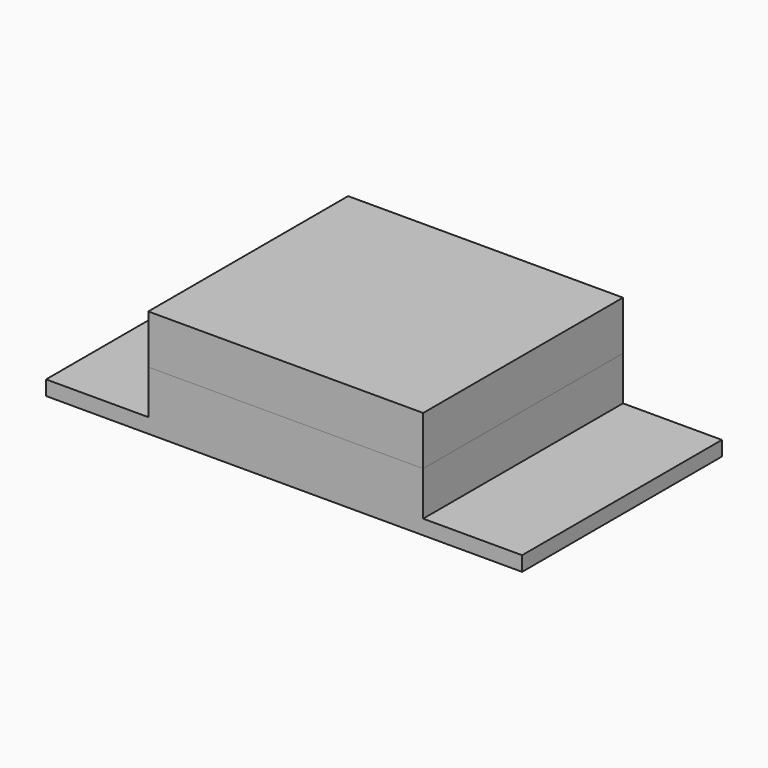
from build123d import *

# Parameters (mm, degrees)
F0_W     = 9.1
F0_H     = 23.5
F1_DEPTH = 1.5
F0_W_2   = 9.4355237663
F0_W_3   = 12.3644762337
F0_H_2   = 11.25
F2_DEPTH = 0.5
F0_W_4   = 12.7
F0_W_5   = 27.0644762337
F0_H_3   = 24.5
F3_DEPTH = 6
F4_DEPTH = 10
F5_W     = 28.0644762337
F5_H     = 25.5
F5_W_2   = 27.0644762337
F5_H_2   = 24.5
F6_DEPTH = 4
F7_W     = 28.0644762337
F7_H     = 25.5
F8_DEPTH = 1


# Not quite as in the source:
# - a feature names something its author has since deleted; it is built from what else it names


with BuildPart() as f1:
    # F0 (on Top) → F1 (new body)
    with BuildSketch(Plane.XY):
        with Locations((18.75, 0)):
            Rectangle(F0_W, F0_H)
        Polygon((24.3, -12.75), (24.3, 12.75), (14.2, 12.75), (14.2, 11.75), (23.3, 11.75), (23.3, -11.75), (14.2, -11.75), (14.2, -12.75), align=None)
    extrude(amount=F1_DEPTH)



with BuildPart() as f1b:
    # F0 (on Top) → F1, piece 2 (new body)
    with BuildSketch(Plane.XY):
        Polygon((-13.8644762337, 11.75), (-13.8644762337, 12.75), (-24.3, 12.75), (-24.3, -12.75), (-13.8644762337, -12.75), (-13.8644762337, -11.75), (-23.3, -11.75), (-23.3, 11.75), align=None)
        with Locations((-18.5822381169, 0)):
            Rectangle(F0_W_2, F0_H)
    extrude(amount=F1_DEPTH)


with BuildPart() as f2:
    # F0 (on Top) → F2 (new body)
    with BuildSketch(Plane.XY):
        with Locations((-6.6822381169, 6.125)):
            Rectangle(F0_W_3, F0_H_2)
    extrude(amount=F2_DEPTH)


with BuildPart() as f2b:
    # F0 (on Top) → F2, piece 2 (new body)
    with BuildSketch(Plane.XY):
        with Locations((6.85, 6.125)):
            Rectangle(F0_W_4, F0_H_2)
    extrude(amount=F2_DEPTH)


with BuildPart() as f2c:
    # F0 (on Top) → F2, piece 3 (new body)
    with BuildSketch(Plane.XY):
        with Locations((-6.6822381169, -6.125)):
            Rectangle(F0_W_3, F0_H_2)
    extrude(amount=F2_DEPTH)


with BuildPart() as f2d:
    # F0 (on Top) → F2, piece 4 (new body)
    with BuildSketch(Plane.XY):
        with Locations((6.85, -6.125)):
            Rectangle(F0_W_4, F0_H_2)
    extrude(amount=F2_DEPTH)


with BuildPart() as f1_1:
    add(f1.part)

    add(f1b.part)  # F3 merges F1b
    # F0 (on Top) → F3 (join)
    with BuildSketch(Plane.XY):
        Polygon((14.2, 11.75), (14.2, 12.75), (-13.8644762337, 12.75), (-13.8644762337, 11.75), (-13.8644762337, -11.75), (-13.8644762337, -12.75), (14.2, -12.75), (14.2, -11.75), align=None)
        with Locations((0.1677618831, 0)):
            Rectangle(F0_W_5, F0_H_3, mode=Mode.SUBTRACT)
    extrude(amount=F3_DEPTH)


    add(f2.part)  # F4 merges F2

    add(f2b.part)  # F4 merges F2b

    add(f2c.part)  # F4 merges F2c

    add(f2d.part)  # F4 merges F2d
    # F0 (on Top) → F4 (join)
    with BuildSketch(Plane.XY):
        with Locations((0.1677618831, 0)):
            Rectangle(F0_W_5, F0_H_3)
        with Locations((-6.6822381169, -6.125)):
            Rectangle(F0_W_3, F0_H_2, mode=Mode.SUBTRACT)
        with Locations((6.85, -6.125)):
            Rectangle(F0_W_4, F0_H_2, mode=Mode.SUBTRACT)
        with Locations((-6.6822381169, 6.125)):
            Rectangle(F0_W_3, F0_H_2, mode=Mode.SUBTRACT)
        with Locations((6.85, 6.125)):
            Rectangle(F0_W_4, F0_H_2, mode=Mode.SUBTRACT)
    extrude(amount=F4_DEPTH)


with BuildPart() as f6:
    # F5 (on face) → F6 (new body)
    with BuildSketch(Plane.XY.offset(6)):
        with Locations((0.1677618831, 0)):
            Rectangle(F5_W, F5_H)
        with Locations((0.1677618831, 0)):
            Rectangle(F5_W_2, F5_H_2, mode=Mode.SUBTRACT)
    extrude(amount=F6_DEPTH)

    # F7 (on face) → F8 (join)
    with BuildSketch(Plane.XY.offset(10)):
        with Locations((0.1677618831, 0)):
            Rectangle(F7_W, F7_H)
    extrude(amount=F8_DEPTH)


solid = Compound([f1_1.part, f6.part])
